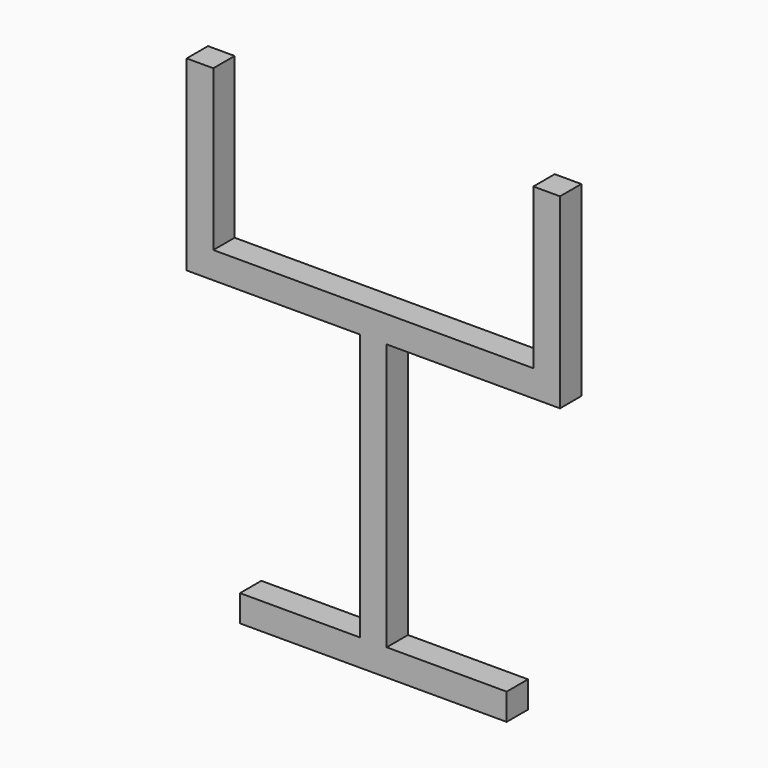
from build123d import *

# Parameters (mm, degrees)
F0_W     = 5
F0_H     = 50
F0_H_2   = 30
F1_DEPTH = 5


# Not quite as in the source:
# - a feature of the source that left no trace in its solid (it failed there, or was rolled back) is left out


with BuildPart() as f1:
    # F0 (on Front) → F1 (new body)
    with BuildSketch(Plane.XZ):
        Polygon((-35, 26.1184218031), (-2.5, 26.1184218031), (2.5, 26.1184218031), (35, 26.1184218031), (35, 31.1184218031), (30, 31.1184218031), (-30, 31.1184218031), (-35, 31.1184218031), align=None)
        with Locations((0, 1.1184218031)):
            Rectangle(F0_W, F0_H)
        Polygon((2.5, -23.8815781969), (-2.5, -23.8815781969), (-25, -23.8815781969), (-25, -28.8815781969), (25, -28.8815781969), (25, -23.8815781969), align=None)
        with Locations((-32.5, 46.1184218031)):
            Rectangle(F0_W, F0_H_2)
        with Locations((32.5, 46.1184218031)):
            Rectangle(F0_W, F0_H_2)
    extrude(amount=F1_DEPTH)


solid = f1.part
